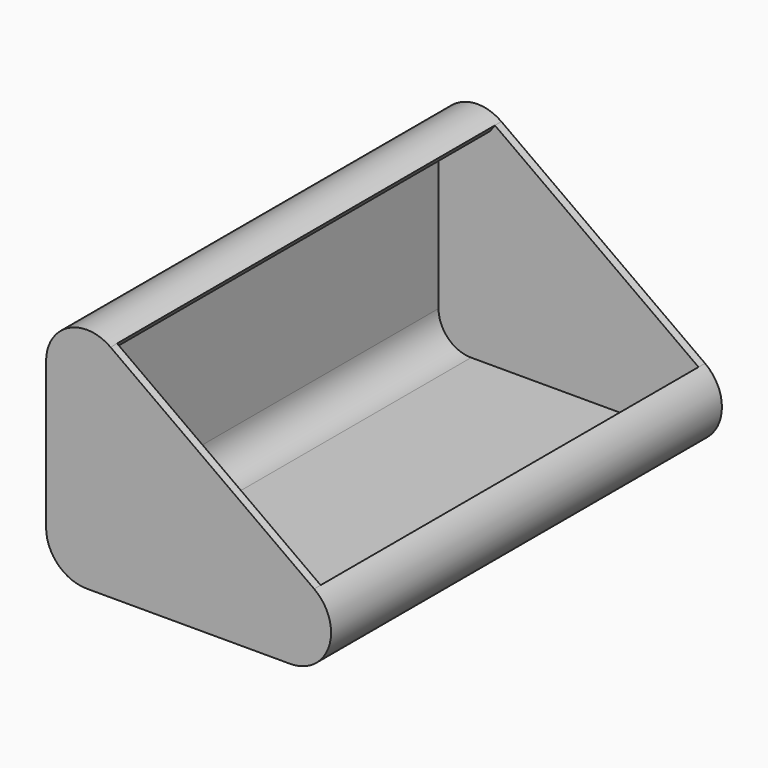
from build123d import *

# Parameters (mm, degrees)
F1_DEPTH      = 127
F1_DEPTH_BACK = 25.4
F3_T          = -2.54


# Not quite as in the source:
# - a feature of the source that left no trace in its solid (it failed there, or was rolled back) is left out
# - a shell that OpenCascade refuses in one call is made with other operations: the cavity is built on its own and cut out


with BuildPart() as f1:
    # F0 (on Front) → F1 (new body, two sides)
    with BuildSketch(Plane.XZ) as f1_sk:
        with BuildLine():
            ThreePointArc((-12.7, 45.72), (0, 33.02), (12.7, 45.72))
            ThreePointArc((12.7, 45.72), (11.3033735945, 51.5099693768), (7.4206700182, 56.0264861364))
            ThreePointArc((7.4206700182, 56.0264861364), (-5.7899693768, 57.0233735945), (-12.7, 45.72))
        make_face()
        with BuildLine():
            ThreePointArc((7.4206700182, 56.0264861364), (11.3033735945, 51.5099693768), (12.7, 45.72))
            ThreePointArc((12.7, 45.72), (0, 33.02), (-12.7, 45.72))
            Line((-12.7, 45.72), (-12.7, 0))
            ThreePointArc((-12.7, 0), (0, 12.7), (12.7, 0))
            ThreePointArc((12.7, 0), (8.9802561211, -8.9802561211), (0, -12.7))
            Line((0, -12.7), (63.5, -12.7))
            ThreePointArc((63.5, -12.7), (51.4131812719, 3.8985655097), (70.9206700182, 10.3064861364))
            Line((70.9206700182, 10.3064861364), (7.4206700182, 56.0264861364))
        make_face()
        with BuildLine():
            ThreePointArc((76.2, 0), (74.8033735945, 5.7899693768), (70.9206700182, 10.3064861364))
            ThreePointArc((70.9206700182, 10.3064861364), (51.4131812719, 3.8985655097), (63.5, -12.7))
            ThreePointArc((63.5, -12.7), (72.4802561211, -8.9802561211), (76.2, 0))
        make_face()
        with BuildLine():
            ThreePointArc((12.7, 0), (0, 12.7), (-12.7, 0))
            ThreePointArc((-12.7, 0), (-8.9802561211, -8.9802561211), (0, -12.7))
            ThreePointArc((0, -12.7), (8.9802561211, -8.9802561211), (12.7, 0))
        make_face()
    extrude(amount=F1_DEPTH)
    extrude(f1_sk.sketch, amount=-F1_DEPTH_BACK)

    # F3: a shell. OpenCascade refuses it in one call, so the cavity is built on its own and cut out:
    # the body offset inwards by the wall thickness, plus a prism from it out through each open face.
    f3_core = offset(f1.part, amount=F3_T, mode=Mode.PRIVATE)
    f3_exits = [f3_core.faces().sort_by_distance(p)[0] for p in [
        (37.686536, -50.8, 31.105189),
    ]]
    add(f3_core, mode=Mode.SUBTRACT)
    extrude(f3_exits, amount=-F3_T, mode=Mode.SUBTRACT)


solid = f1.part
